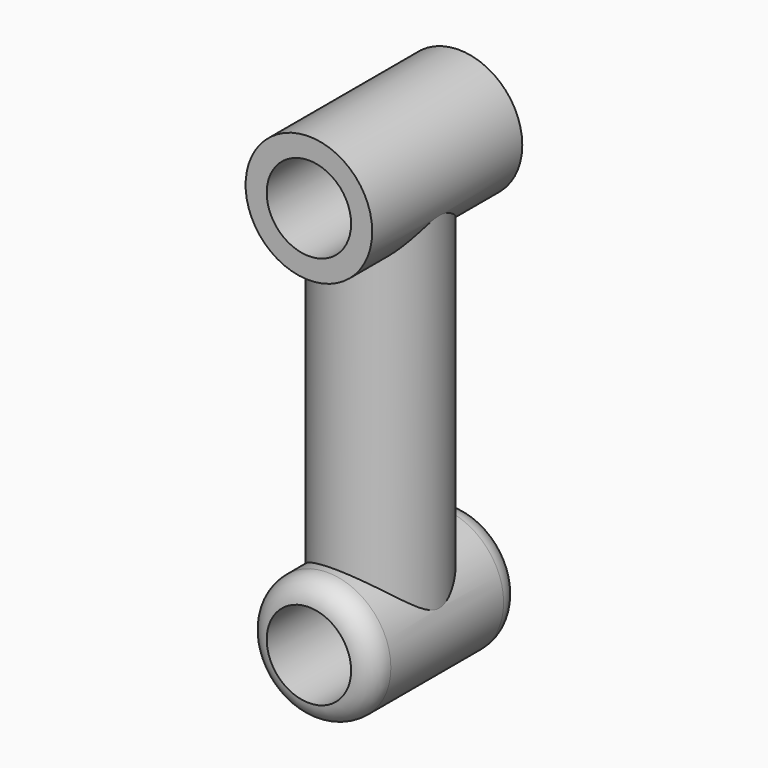
from build123d import *

# Parameters (mm, degrees)
F0_R     = 2.7
F0_R_2   = 1.8
F1_DEPTH = 8
F2_R     = 2.5
F3_DEPTH = 16
F4_DEPTH = 25
F5_R     = 2.7
F5_R_2   = 1.8
F6_DEPTH = 8
F7_DEPTH = 25


# Not quite as in the source:
# - a fillet or chamfer that OpenCascade refuses, or shapes differently, is made with other operations: its cross-section is extruded or revolved along the edge and cut away or added


with BuildPart() as f1:
    # F0 (on Front) → F1 (new body)
    with BuildSketch(Plane.XZ):
        with Locations((0, 0.773217123)):
            Circle(F0_R)
        with Locations((0, 0.773217123)):
            Circle(F0_R_2, mode=Mode.SUBTRACT)
    extrude(amount=F1_DEPTH)

    # F2 (on Top) → F3 (join)
    with BuildSketch(Plane.XY):
        with Locations((0, -4.1738846339)):
            Circle(F2_R)
    extrude(amount=-F3_DEPTH)

    # F0 (on Front) → F4 (cut)
    with BuildSketch(Plane.XZ):
        with Locations((0, 0.773217123)):
            Circle(F0_R_2)
    extrude(amount=F4_DEPTH, mode=Mode.SUBTRACT)

    # F5 (on Front) → F6 (join, through all)
    with BuildSketch(Plane.XZ):
        with Locations((0, -16.0034396241)):
            Circle(F5_R)
        with Locations((0, -16.0034396241)):
            Circle(F5_R_2, mode=Mode.SUBTRACT)
    extrude(amount=F6_DEPTH)

    # F5 (on Front) → F7 (cut)
    with BuildSketch(Plane.XZ):
        with Locations((0, -16.0034396241)):
            Circle(F5_R_2)
    extrude(amount=F7_DEPTH, mode=Mode.SUBTRACT)

    # F8: fillet of radius 1 on 1 edges, made by hand

    # F8_s1 → F8_t2 (revolve, cut)
    with BuildSketch(Plane.XY.offset(-16.0034396241)):
        with BuildLine():
            ThreePointArc((2.7, -0.9949874371), (2.4416198487, -0.3241670439), (1.8, 0))
            Line((1.8, 0), (2.7, 0))
            Line((2.7, 0), (2.7, -0.9949874371))
        make_face()
    revolve(axis=Axis((0, 0, -16.0034396241), (0, -1, 0)), mode=Mode.SUBTRACT)

    # F9: fillet of radius 1 on 1 edges, made by hand

    # F9_s1 → F9_t2 (revolve, cut)
    with BuildSketch(Plane.XY.offset(-16.0034396241)):
        with BuildLine():
            ThreePointArc((2.7, -7.0050125629), (2.4416198487, -7.6758329561), (1.8, -8))
            Line((1.8, -8), (2.7, -8))
            Line((2.7, -8), (2.7, -7.0050125629))
        make_face()
    revolve(axis=Axis((0, -8, -16.0034396241), (0, -1, 0)), mode=Mode.SUBTRACT)


solid = f1.part
